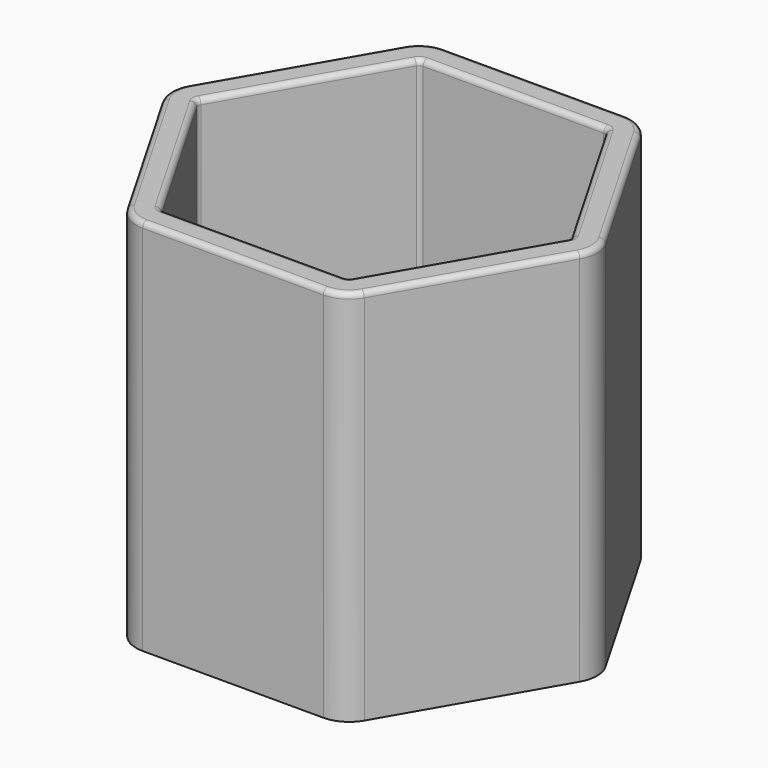
from build123d import *

# Parameters (mm, degrees)
F1_DEPTH        = 70
F3_DEPTH        = 5
F4_R            = 2.5
F5_DEPTH        = 5
F5_COPIES_COUNT = 4
F7_R            = 2.5
F8_DEPTH        = 5
F9_R            = 6
F10_R           = 1
F11_R           = 1


# Not quite as in the source:
# - a pattern or mirror of a feature is missing from the dataset's text; its kind, count and spacing are read off the source's solid


with BuildPart() as f1:
    # F0 (on Top) → F1 (new body)
    with BuildSketch(Plane.XY):
        Polygon((20.2072594216, 35), (-20.2072594216, 35), (-40.4145188433, 0), (-20.2072594216, -35), (20.2072594216, -35), (40.4145188433, 0), align=None)
        Polygon((-17.3205080757, -30), (-34.6410161514, 0), (-17.3205080757, 30), (17.3205080757, 30), (34.6410161514, 0), (17.3205080757, -30), align=None, mode=Mode.SUBTRACT)
    extrude(amount=F1_DEPTH)

    # F2 (on face) → F3 (join)
    with BuildSketch(Plane(origin=(0, 0, 0), x_dir=(1, 0, 0), z_dir=(0, 0, -1))):
        Polygon((-20.2072594216, 35), (-40.4145188433, 0), (-20.2072594216, -35), (20.2072594216, -35), (40.4145188433, 0), (20.2072594216, 35), align=None)
    extrude(amount=-F3_DEPTH)

    # F4 (on face) → F5 (cut, through all)
    with BuildSketch(Plane.XY.offset(5)):
        with Locations((0, 26)):
            Circle(F4_R)
        with Locations((4.4861967818, 16.7427143223)):
            Circle(F4_R)
        with Locations((0, 8.6666666667)):
            Circle(F4_R)
        with Locations((12.2565175406, 12.2565175406)):
            Circle(F4_R)
        with Locations((9.9497692415, 24.0208678453)):
            Circle(F4_R)
        with Locations((24.0208678453, 9.9497692415)):
            Circle(F4_R)
        with Locations((16.7427143223, 4.4861967818)):
            Circle(F4_R)
        with Locations((18.3847763109, 18.3847763109)):
            Circle(F4_R)
    f5 = extrude(amount=-F5_DEPTH, mode=Mode.SUBTRACT)

    # F5_copies: F5 ×4 about axis
    f5_copies_axis = Axis((0, 0, 0), (0, 0, 1))
    for i in range(1, F5_COPIES_COUNT):
        add(f5.rotate(f5_copies_axis, i * 360 / F5_COPIES_COUNT), mode=Mode.SUBTRACT)

    # F7 (on face) → F8 (cut, through all)
    with BuildSketch(Plane.XY.offset(5)):
        Circle(F7_R)
    extrude(amount=-F8_DEPTH, mode=Mode.SUBTRACT)

    # F9
    f9_edges = [f1.edges().sort_by_distance(p)[0] for p in [
        (-20.207259, 35, 35),
        (-40.414519, 0, 35),
        (-20.207259, -35, 35),
        (20.207259, -35, 35),
        (40.414519, 0, 35),
        (20.207259, 35, 35),
    ]]
    fillet(f9_edges, radius=F9_R)

    # F10
    f10_edges = [f1.edges().sort_by_distance(p)[0] for p in [
        (-17.320508, 30, 37.5),
        (17.320508, 30, 37.5),
        (34.641016, 0, 37.5),
        (17.320508, -30, 37.5),
        (-17.320508, -30, 37.5),
        (-34.641016, 0, 37.5),
        (-25.980762, 15, 5),
        (-25.980762, -15, 5),
        (0, -30, 5),
        (25.980762, -15, 5),
        (25.980762, 15, 5),
        (0, 30, 5),
    ]]
    fillet(f10_edges, radius=F10_R)

    # F11
    f11_edges = [f1.edges().sort_by_distance(p)[0] for p in [
        (-25.980762, -15, 70),
        (-17.243158, -29.866025, 70),
        (-34.486316, 0, 70),
        (0, -30, 70),
        (-25.980762, 15, 70),
        (17.243158, -29.866025, 70),
        (-17.243158, 29.866025, 70),
        (25.980762, -15, 70),
        (0, 30, 70),
        (34.486316, 0, 70),
        (17.243158, 29.866025, 70),
        (25.980762, 15, 70),
        (0, 35, 70),
        (19.743158, 34.196152, 70),
        (-19.743158, 34.196152, 70),
        (30.310889, 17.5, 70),
        (-30.310889, 17.5, 70),
        (39.486316, 0, 70),
        (-39.486316, 0, 70),
        (30.310889, -17.5, 70),
        (-30.310889, -17.5, 70),
        (19.743158, -34.196152, 70),
        (-19.743158, -34.196152, 70),
        (0, -35, 70),
    ]]
    fillet(f11_edges, radius=F11_R)


solid = f1.part
